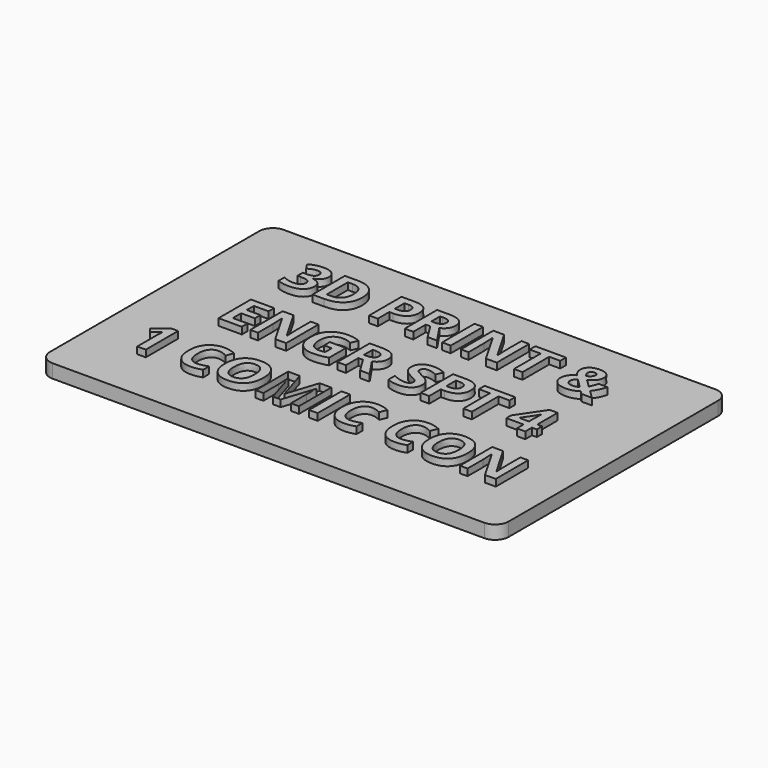
from build123d import *

# Parameters (mm, degrees)
F1_DEPTH     = 2.54
F2_TEXT_SIZE = 10.5833333333
F3_DEPTH     = 1.27


# Not quite as in the source:
# - Text() gives the source's letters only with a copy of the font that has no kerning and outlines rounded to 1/6400 em; it was checked with that copy


with BuildPart() as f1:
    # F0 (on Top) → F1 (new body)
    with BuildSketch(Plane.XY):
        with BuildLine():
            ThreePointArc((42.8625, 24.4475), (42.1185512242, 26.2435512242), (40.3225, 26.9875))
            Line((40.3225, 26.9875), (-40.3225, 26.9875))
            ThreePointArc((-40.3225, 26.9875), (-42.1185512242, 26.2435512242), (-42.8625, 24.4475))
            Line((-42.8625, 24.4475), (-42.8625, -24.4475))
            ThreePointArc((-42.8625, -24.4475), (-42.1185512242, -26.2435512242), (-40.3225, -26.9875))
            Line((-40.3225, -26.9875), (40.3225, -26.9875))
            ThreePointArc((40.3225, -26.9875), (42.1185512242, -26.2435512242), (42.8625, -24.4475))
            Line((42.8625, -24.4475), (42.8625, 24.4475))
        make_face()
    extrude(amount=F1_DEPTH)

    # F2 (on face) → F3 (join)
    with BuildSketch(Plane.XY.offset(2.54)):
        with Locations((-29.7424739583, 11.7475)):
            Text('3D PRINT &', F2_TEXT_SIZE, font='Open Sans', font_style=FontStyle.BOLD, text_align=(TextAlign.LEFT, TextAlign.BOTTOM))
        with Locations((-29.7424739583, -2.6458333333)):
            Text('ENGR SPT 4', F2_TEXT_SIZE, font='Open Sans', font_style=FontStyle.BOLD, text_align=(TextAlign.LEFT, TextAlign.BOTTOM))
        with Locations((-35.2425, -17.0391666667)):
            Text('1 COMIC CON', F2_TEXT_SIZE, font='Open Sans', font_style=FontStyle.BOLD, text_align=(TextAlign.LEFT, TextAlign.BOTTOM))
    extrude(amount=F3_DEPTH)


solid = f1.part
